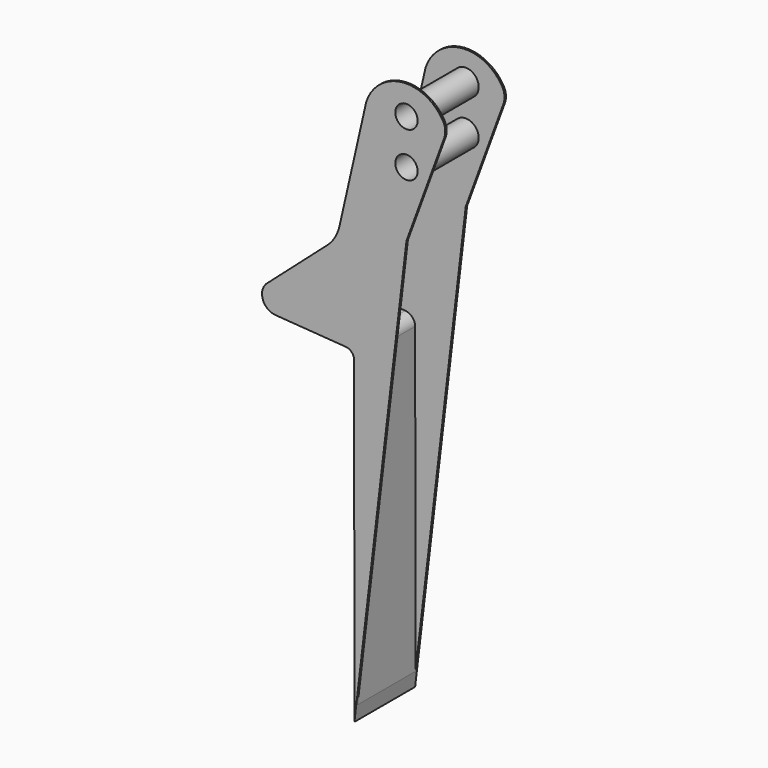
from build123d import *

# Parameters (mm, degrees)
F0_R     = 2.5
F1_DEPTH = 17
F2_T     = 0.4


# Not quite as in the source:
# - a shell that OpenCascade refuses in one call is made with other operations: the cavity is built on its own and cut out


with BuildPart() as f1:
    # F0 (on Front) → F1 (new body)
    with BuildSketch(Plane.XZ):
        with BuildLine():
            ThreePointArc((8.4418530872, -1.5193999292), (8.6686009191, 0.2448895048), (8.1079887938, 1.933038145))
            ThreePointArc((8.1079887938, 1.933038145), (-1.0644623598, 6.4400537212), (-9, 0))
            Line((-9, 0), (-14.990051355, -26.4365585686))
            ThreePointArc((-14.990051355, -26.4365585686), (-16.0266215588, -29.0388056628), (-17.8130271161, -31.1963326989))
            Line((-17.8130271161, -31.1963326989), (-31.2685862961, -43.0686485372))
            ThreePointArc((-31.2685862961, -43.0686485372), (-32.0681766379, -44.1518925803), (-32.3514207584, -45.4681505868))
            Line((-32.3514207584, -45.4681505868), (-32.3514207584, -45.4984797908))
            ThreePointArc((-32.3514207584, -45.4984797908), (-31.4935858742, -47.678906944), (-29.3800066519, -48.6903050507))
            Line((-29.3800066519, -48.6903050507), (-13.5882116102, -49.8212509157))
            ThreePointArc((-13.5882116102, -49.8212509157), (-12.2679323329, -50.4526148934), (-11.7310788719, -51.8140649305))
            Line((-11.7310788719, -51.8140649305), (-11.6569881297, -123.1658389017))
            Line((-11.6569881297, -123.1658389017), (0, -24.5))
            Line((0, -24.5), (8.4418530872, -1.5193999292))
        make_face()
        with Locations((0, -10)):
            Circle(F0_R, mode=Mode.SUBTRACT)
        Circle(F0_R, mode=Mode.SUBTRACT)
    extrude(amount=F1_DEPTH)

    # F2: shell of thickness 0.4, made by hand


with BuildPart() as f2_core1:
    # F2_t2: copy of F1
    add(f1.part)

    # the walls: a layer under each face that stays
    f2_faces = [f2_core1.faces().sort_by_distance(p)[0] for p in [
        (-16.0266215588, -8.5, -29.0388056628),
        (-24.5408067061, -8.5, -37.1324906181),
        (-32.0681766379, -8.5, -44.1518925803),
        (-32.3514207584, -8.5, -45.4833151888),
        (-31.4935858742, -8.5, -47.678906944),
        (-21.484109131, -8.5, -49.2557779832),
        (-12.2679323329, -8.5, -50.4526148934),
        (-11.6940335008, -8.5, -87.4899519161),
        (-2.5, -8.5, -10),
        (-2.5, -8.5, 0),
        (-11.8321233546, 0, -15.1109731503),
        (-11.8321233546, -17, -15.1109731503),
    ]]
    thicken(f2_faces, amount=-F2_T, mode=Mode.SUBTRACT)


with BuildPart() as f1_1:
    add(f1.part)

    # what is left inside the walls is the cavity
    f2_cavity = [f2_core1.part.solids().sort_by_distance(p)[0] for p in [
        (-5.634209, -11.2, -72.154379),
    ]]
    add(f2_cavity, mode=Mode.SUBTRACT)


solid = f1_1.part
